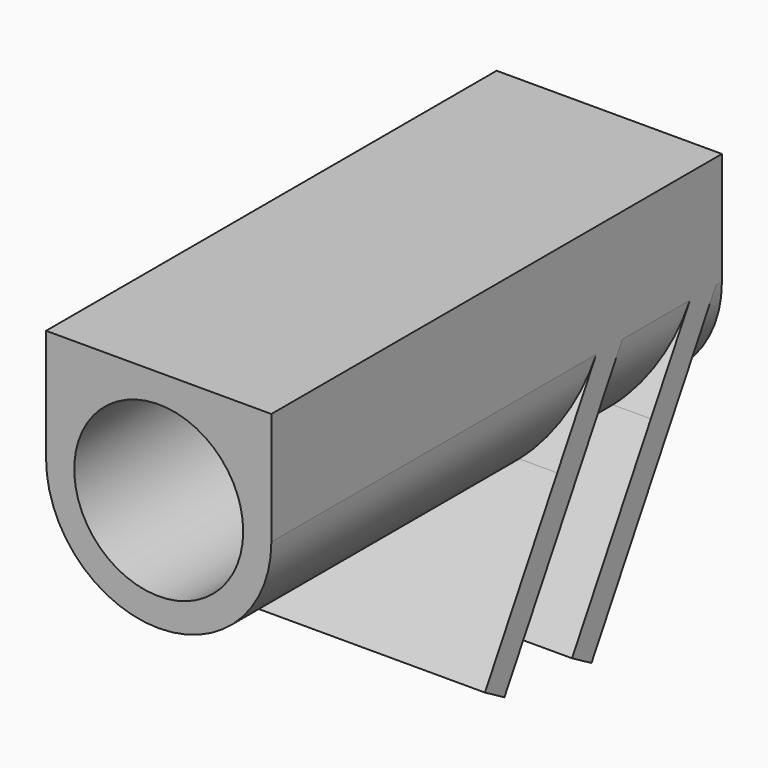
from build123d import *

# Parameters (mm, degrees)
F0_R          = 3
F1_DEPTH      = 20
F3_DEPTH      = 4
F3_DEPTH_BACK = 4
F6_DEPTH      = 1
F9_DEPTH      = 1
F10_DEPTH     = 20


with BuildPart() as f1:
    # F0 (on Front) → F1 (new body)
    with BuildSketch(Plane.XZ):
        with BuildLine():
            ThreePointArc((-4, 0), (0, -4), (4, 0))
            ThreePointArc((4, 0), (2.8284271247, 2.8284271247), (0, 4))
            ThreePointArc((0, 4), (-2.8284271247, 2.8284271247), (-4, 0))
        make_face()
        Circle(F0_R, mode=Mode.SUBTRACT)
    extrude(amount=F1_DEPTH)

    # F2 (on Right) → F3 (join, two sides)
    with BuildSketch(Plane.YZ) as f3_sk:
        Polygon((-5.7886751346, -9.5621778265), (-2, -3), (-3.1547005384, -3), (-6.6547005384, -9.0621778265), align=None)
        Polygon((-9.6547005384, -9.0621778265), (-6.1547005384, -3), (-7.3094010768, -3), (-10.5207259422, -8.5621778265), align=None)
    extrude(amount=F3_DEPTH)
    extrude(f3_sk.sketch, amount=-F3_DEPTH_BACK)

    # F5 (on offset) → F6 (join)
    with BuildSketch(Plane(origin=(0, -0.2009618943, 0.1160254038), x_dir=(-1, 0, 0), z_dir=(0, 0.8660254038, -0.5))):
        Polygon((4, -5), (4, 0), (2, -5), align=None)
        Polygon((-2, -5), (-4, 0), (-4, -5), align=None)
    extrude(amount=-F6_DEPTH)

    # F8 (on offset) → F9 (join)
    with BuildSketch(Plane(origin=(0, -3.3169872981, 1.9150635095), x_dir=(-1, 0, 0), z_dir=(0, 0.8660254038, -0.5))):
        Polygon((4, -7), (4, -2), (2, -7), align=None)
        Polygon((-4, -7), (-2, -7), (-4, -2), align=None)
    extrude(amount=-F9_DEPTH)

    # F0 (on Front) → F10 (join)
    with BuildSketch(Plane.XZ):
        with BuildLine():
            ThreePointArc((-4, 0), (0, -4), (4, 0))
            ThreePointArc((4, 0), (2.8284271247, 2.8284271247), (0, 4))
            ThreePointArc((0, 4), (-2.8284271247, 2.8284271247), (-4, 0))
        make_face()
        Circle(F0_R, mode=Mode.SUBTRACT)
        with BuildLine():
            ThreePointArc((0, 4), (2.8284271247, 2.8284271247), (4, 0))
            Line((4, 0), (4, 4))
            Line((4, 4), (0, 4))
        make_face()
        with BuildLine():
            ThreePointArc((-4, 0), (-2.8284271247, 2.8284271247), (0, 4))
            Line((0, 4), (-4, 4))
            Line((-4, 4), (-4, 0))
        make_face()
    extrude(amount=F10_DEPTH)


solid = f1.part
